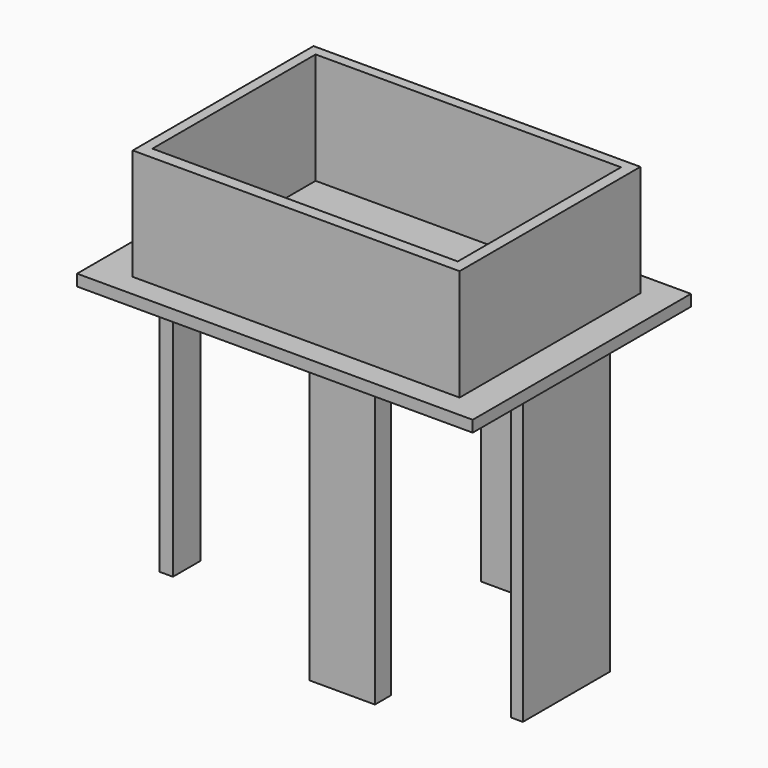
from build123d import *

# Parameters (mm, degrees)
F0_W     = 132.1772886384
F0_H     = 91.3944654167
F0_W_2   = 123.5
F0_H_2   = 82.5
F1_DEPTH = 45
F2_W     = 160
F2_H     = 110.3064134685
F3_DEPTH = 4.6
F4_W     = 26.40013583
F4_H     = 8.1236897111
F4_H_2   = 8.12
F5_DEPTH = 115
F6_W     = 4.7950819135
F6_H     = 44.0778695047
F7_DEPTH = 115
F8_W     = 5.5164026618
F8_H     = 13.8319674879
F9_DEPTH = 115


# Not quite as in the source:
# - the program builds the solid bodies; features that only make, move or delete a surface that nothing else refers to are left out


with BuildPart() as f1:
    # F0 (on Top) → F1 (new body)
    with BuildSketch(Plane.XY):
        with Locations((-0.5622557336, 4.6925004572)):
            Rectangle(F0_W, F0_H)
        with Locations((-0.8209000528, 5.0862303376)):
            Rectangle(F0_W_2, F0_H_2, mode=Mode.SUBTRACT)
    extrude(amount=F1_DEPTH)

    # F2 (on Top) → F3 (join)
    with BuildSketch(Plane.XY):
        with Locations((-1.752063632, 4.8872958869)):
            Rectangle(F2_W, F2_H)
    extrude(amount=-F3_DEPTH)

    # F4 (on face) → F5 (join)
    with BuildSketch(Plane(origin=(0, 0, -4.6), x_dir=(1, 0, 0), z_dir=(0, 0, -1))):
        with Locations((19.0718499944, 38.1715348911)):
            Rectangle(F4_W, F4_H)
        with Locations((19.0718499944, -48.4503099644)):
            Rectangle(F4_W, F4_H_2)
    extrude(amount=F5_DEPTH)

    # F6 (on face) + F4 (on face) → F7 (join)
    with BuildSketch(Plane(origin=(0, 0, -4.6), x_dir=(1, 0, 0), z_dir=(0, 0, -1))):
        with Locations((73.7704820931, 0.2766400576)):
            Rectangle(F6_W, F6_H)
    with BuildSketch(Plane(origin=(0, 0, -4.6), x_dir=(1, 0, 0), z_dir=(0, 0, -1))):
        with Locations((19.0718499944, 38.1715348911)):
            Rectangle(F4_W, F4_H)
        with Locations((19.0718499944, -48.4503099644)):
            Rectangle(F4_W, F4_H_2)
    extrude(amount=F7_DEPTH)

    # F8 (on face) → F9 (join)
    with BuildSketch(Plane(origin=(0, 0, -4.6), x_dir=(1, 0, 0), z_dir=(0, 0, -1))):
        with Locations((-74.8852601945, 6.915983744)):
            Rectangle(F8_W, F8_H)
    extrude(amount=F9_DEPTH)


solid = f1.part
